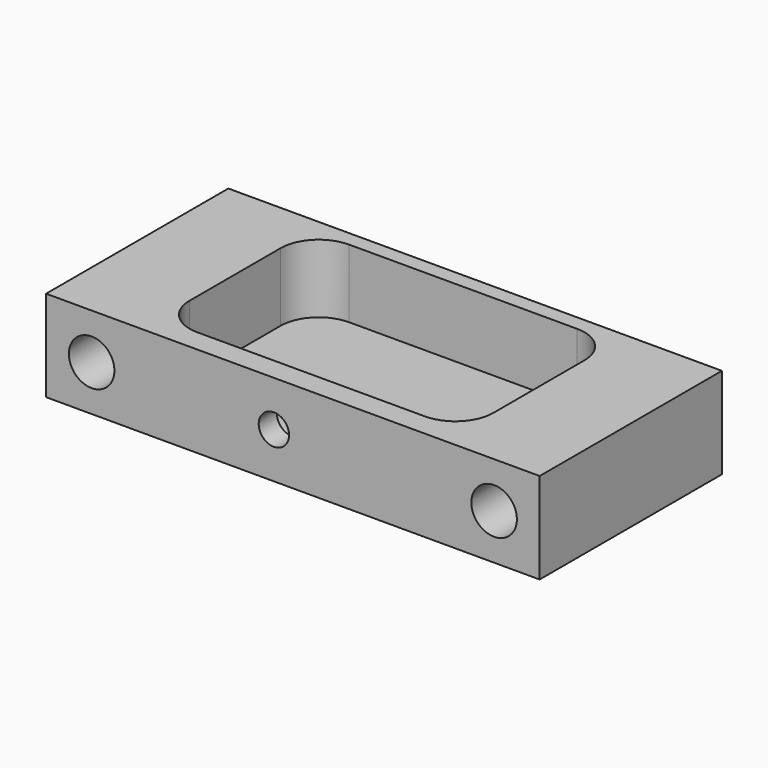
from build123d import *

# Parameters (mm, degrees)
F0_W     = 65
F0_H     = 30
F1_DEPTH = 12
F4_D     = 6
F5_D     = 6
F6_W     = 40
F6_H     = 25
F7_DEPTH = 9
F8_R     = 5
F9_D     = 4
F9_DEPTH = 7
F9_TIP   = 1.2017212381


# Not quite as in the source:
# - a feature names something its author has since deleted; it is built from what else it names


with BuildPart() as f1:
    # F0 (on Top) → F1 (new body)
    with BuildSketch(Plane.XY):
        with Locations((10.1498100485, -9.411229075)):
            Rectangle(F0_W, F0_H)
    extrude(amount=F1_DEPTH)

    # F4 (through all)
    with Locations(Plane.XZ.offset(24.411229075)):
        with Locations((36.6498100485, 6)):
            Hole(F4_D / 2)

    # F5 (through all)
    with Locations(Plane.XZ.offset(24.411229075)):
        with Locations((-16.3501899515, 6)):
            Hole(F5_D / 2)

    # F6 (on face) → F7 (cut)
    with BuildSketch(Plane.XY.offset(12)):
        with Locations((10.1498100485, -8.911229075)):
            Rectangle(F6_W, F6_H)
    extrude(amount=-F7_DEPTH, mode=Mode.SUBTRACT)

    # F8
    f8_edges = [f1.edges().sort_by_distance(p)[0] for p in [
        (-9.85019, 3.588771, 7.5),
        (-9.85019, -21.411229, 7.5),
        (30.14981, 3.588771, 7.5),
        (30.14981, -21.411229, 7.5),
    ]]
    fillet(f8_edges, radius=F8_R)

    # F9
    with Locations(Plane.XZ.offset(24.411229075)):
        with Locations((7.6498100485, 6)):
            Hole(F9_D / 2, depth=F9_DEPTH)
            with Locations((0, 0, -(F9_DEPTH + F9_TIP / 2))):  # 118° drill point
                Cone(0, F9_D / 2, F9_TIP, mode=Mode.SUBTRACT)


solid = f1.part
